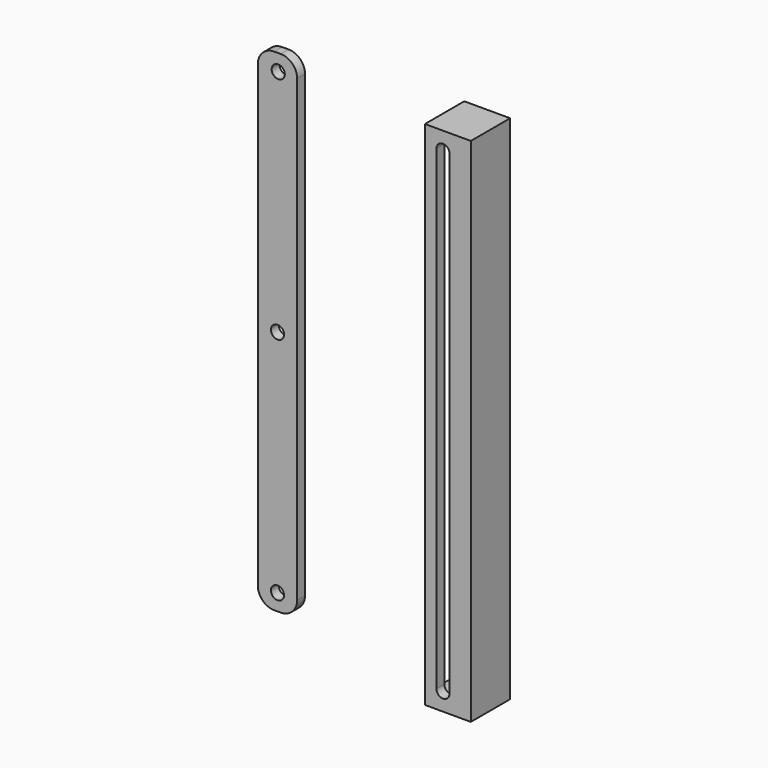
from build123d import *

# Parameters (mm, degrees)
F0_R      = 2
F1_DEPTH  = 3
F2_DEPTH  = 3
F3_DEPTH  = 15
F4_W      = 9
F4_H      = 3
F5_DEPTH  = 150
F6_W      = 9
F6_H      = 9
F7_DEPTH  = 3
F8_START  = -153
F7_FACE_W = 12
F7_FACE_H = 15
F8_DEPTH  = 3
F9_DEPTH  = 15
F10_DEPTH = 2


with BuildPart() as f1:
    # F0 (on Front) → F1 (new body)
    with BuildSketch(Plane.XZ):
        with BuildLine():
            Line((-36.8372175097, 75.0188916922), (-38.8372175097, 75.0188916922))
            ThreePointArc((-38.8372175097, 75.0188916922), (-42.3727514157, 73.5544255981), (-43.8372175097, 70.0188916922))
            Line((-43.8372175097, 70.0188916922), (-43.8372175097, -69.9811083078))
            ThreePointArc((-43.8372175097, -69.9811083078), (-42.3727514157, -73.5166422138), (-38.8372175097, -74.9811083078))
            Line((-38.8372175097, -74.9811083078), (-36.8372175097, -74.9811083078))
            ThreePointArc((-36.8372175097, -74.9811083078), (-33.3016836038, -73.5166422138), (-31.8372175097, -69.9811083078))
            Line((-31.8372175097, -69.9811083078), (-31.8372175097, 70.0188916922))
            ThreePointArc((-31.8372175097, 70.0188916922), (-33.3016836038, 73.5544255981), (-36.8372175097, 75.0188916922))
        make_face()
        with Locations((-37.8372175097, -69.9811083078)):
            Circle(F0_R, mode=Mode.SUBTRACT)
        with Locations((-37.8372175097, 0.0094458461)):
            Circle(F0_R, mode=Mode.SUBTRACT)
        with Locations((-37.616844722, 69.9996530654)):
            Circle(F0_R, mode=Mode.SUBTRACT)
    extrude(amount=F1_DEPTH)


with BuildPart() as f2:
    # F0 (on Front) → F2 (new body)
    with BuildSketch(Plane.XZ):
        Polygon((30.7263619155, 75.5200837851), (27.7263619155, 75.5200837851), (27.7263619155, -74.4799162149), (30.7263619155, -74.4799162149), (30.7263619155, -69.9799162149), (30.7263619155, 70.0200837851), align=None)
        Polygon((27.7263619155, 75.5200837851), (24.2263619155, 75.5200837851), (24.2263619155, 73.0200837851), (24.2263619155, -71.9799162149), (24.2263619155, -74.4799162149), (27.7263619155, -74.4799162149), align=None)
        with BuildLine():
            Line((24.2263619155, 75.5200837851), (20.2263619155, 75.5200837851))
            Line((20.2263619155, 75.5200837851), (20.2263619155, 73.0200837851))
            ThreePointArc((20.2263619155, 73.0200837851), (22.2263619155, 75.0200837851), (24.2263619155, 73.0200837851))
            Line((24.2263619155, 73.0200837851), (24.2263619155, 75.5200837851))
        make_face()
        with BuildLine():
            Line((20.2263619155, -71.9799162149), (20.2263619155, -74.4799162149))
            Line((20.2263619155, -74.4799162149), (24.2263619155, -74.4799162149))
            Line((24.2263619155, -74.4799162149), (24.2263619155, -71.9799162149))
            ThreePointArc((24.2263619155, -71.9799162149), (22.2263619155, -73.9799162149), (20.2263619155, -71.9799162149))
        make_face()
        Polygon((18.7263619155, 75.5200837851), (18.7263619155, 70.5200837851), (18.7263619155, -69.4799162149), (18.7263619155, -74.4799162149), (20.2263619155, -74.4799162149), (20.2263619155, -71.9799162149), (20.2263619155, 73.0200837851), (20.2263619155, 75.5200837851), align=None)
    extrude(amount=F2_DEPTH)

    # F0 (on Front) → F3 (join)
    with BuildSketch(Plane.XZ):
        Polygon((30.7263619155, 75.5200837851), (27.7263619155, 75.5200837851), (27.7263619155, -74.4799162149), (30.7263619155, -74.4799162149), (30.7263619155, -69.9799162149), (30.7263619155, 70.0200837851), align=None)
    extrude(amount=F3_DEPTH)

    # F4 (on face) → F5 (join, through all)
    with BuildSketch(Plane.XY.offset(75.5200837851)):
        with Locations((23.2263619155, -13.5)):
            Rectangle(F4_W, F4_H)
    extrude(amount=-F5_DEPTH)

    # F6 (on face) → F7 (join)
    with BuildSketch(Plane.XY.offset(75.5200837851)):
        Polygon((18.7263619155, 0), (18.7263619155, -3), (27.7263619155, -3), (27.7263619155, -12), (18.7263619155, -12), (18.7263619155, -15), (30.7263619155, -15), (30.7263619155, 0), align=None)
        with Locations((23.2263619155, -7.5)):
            Rectangle(F6_W, F6_H)
    extrude(amount=F7_DEPTH)

    # F7_face (on face) → F8 (join)
    with BuildSketch(Plane(origin=(24.7263619155, -7.5, 78.5200837851), x_dir=(1, 0, 0), z_dir=(0, 0, 1)).offset(F8_START)):
        Rectangle(F7_FACE_W, F7_FACE_H)
    extrude(amount=-F8_DEPTH)

    # F0 (on Front) → F9 (cut, through all)
    with BuildSketch(Plane.XZ):
        with BuildLine():
            ThreePointArc((24.2263619155, 73.0200837851), (22.2263619155, 75.0200837851), (20.2263619155, 73.0200837851))
            Line((20.2263619155, 73.0200837851), (20.2263619155, -71.9799162149))
            ThreePointArc((20.2263619155, -71.9799162149), (22.2263619155, -73.9799162149), (24.2263619155, -71.9799162149))
            Line((24.2263619155, -71.9799162149), (24.2263619155, 73.0200837851))
        make_face()
    extrude(amount=F9_DEPTH, mode=Mode.SUBTRACT)

    # F10 (add): a face of the model
    f10_faces = [f2.faces().sort_by_distance(p)[0] for p in [
        (18.7263619155, -1.5671949464, 0.5200837851),
    ]]
    extrude(f10_faces, amount=F10_DEPTH)


solid = Compound([f1.part, f2.part])
